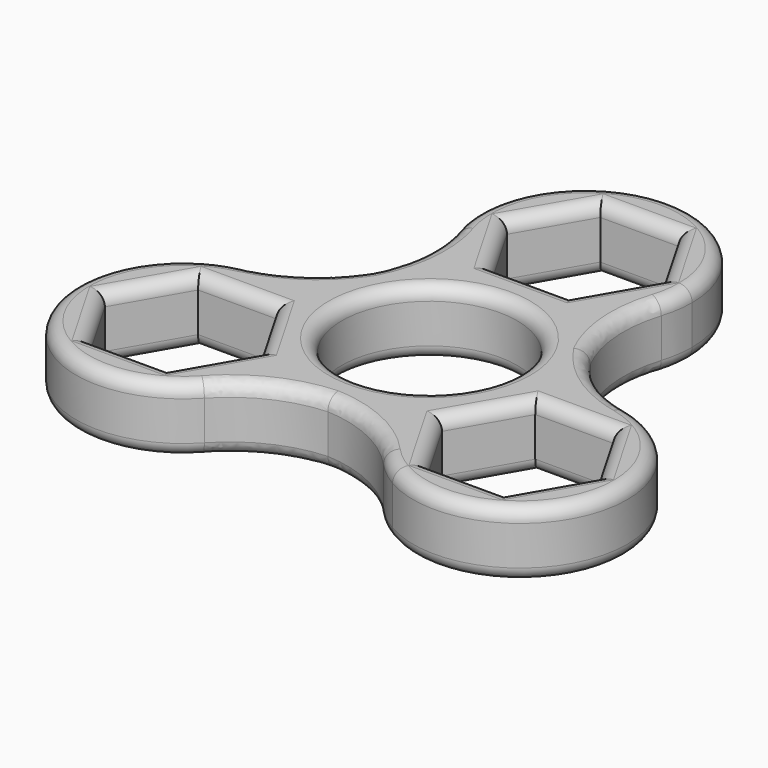
from build123d import *

# Parameters (mm, degrees)
F3_DEPTH = 5
F4_R     = 10
F5_COUNT = 3
F6_R     = 1


# Not quite as in the source:
# - a feature of the source that left no trace in its solid (it failed there, or was rolled back) is left out


with BuildPart() as f3:
    # F2 (on Top) → F3 (new body)
    with BuildSketch(Plane.XY):
        with BuildLine():
            ThreePointArc((8.175, 14.875), (-3.6420010923, 22.193910646), (-4.9299426406, 8.3537815126))
            ThreePointArc((-4.9299426406, 8.3537815126), (-2.5552220381, 9.3573949546), (0, 9.7))
            ThreePointArc((0, 9.7), (2.5552220381, 9.3573949546), (4.9299426406, 8.3537815126))
            ThreePointArc((4.9299426406, 8.3537815126), (7.318910646, 11.2329989077), (8.175, 14.875))
        make_face()
        Polygon((2.9877876431, 9.7), (0, 9.7), (-2.9877876431, 9.7), (-5.9755752861, 14.875), (-2.9877876431, 20.05), (2.9877876431, 20.05), (5.9755752861, 14.875), align=None, mode=Mode.SUBTRACT)
        with BuildLine():
            ThreePointArc((-4.9299426406, 8.3537815126), (-2.5999676792, 7.1244649819), (0, 6.7))
            ThreePointArc((0, 6.7), (2.5999676792, 7.1244649819), (4.9299426406, 8.3537815126))
            ThreePointArc((4.9299426406, 8.3537815126), (2.5552220381, 9.3573949546), (0, 9.7))
            ThreePointArc((0, 9.7), (-2.5552220381, 9.3573949546), (-4.9299426406, 8.3537815126))
        make_face()
        with BuildLine():
            ThreePointArc((4.9299426406, 8.3537815126), (2.5999676792, 7.1244649819), (0, 6.7))
            ThreePointArc((0, 6.7), (-2.5999676792, 7.1244649819), (-4.9299426406, 8.3537815126))
            ThreePointArc((-4.9299426406, 8.3537815126), (-4.8098625961, -8.4234922572), (9.7, 0))
            ThreePointArc((9.7, 0), (8.4234922572, 4.8098625961), (4.9299426406, 8.3537815126))
        make_face()
        with BuildLine():
            ThreePointArc((0, 6.7), (4.7376154339, 4.737615434), (6.7, 0))
            ThreePointArc((6.7, 0), (-4.7376154339, -4.737615434), (0, 6.7))
        make_face(mode=Mode.SUBTRACT)
    extrude(amount=F3_DEPTH)

    # F4
    f4_edges = [f3.edges().sort_by_distance(p)[0] for p in [
        (4.929943, 8.353782, 2.5),
        (-4.929943, 8.353782, 2.5),
    ]]
    fillet(f4_edges, radius=F4_R)

    # F5: F3 ×3 about axis
    f5_axis = Axis((0, 0, 0), (0, 0, -1))


with BuildPart() as f3_1:
    add(f3.part)
    for i in range(1, F5_COUNT):
        add(f3.part.rotate(f5_axis, i * 360 / F5_COUNT))

    # F6
    f6_edges = [f3_1.edges().sort_by_distance(p)[0] for p in [
        (7.357055, 8.567839, 5),
        (0, 23.05, 5),
        (-7.357055, 8.56784, 5),
        (-11.098494, 2.087477, 5),
        (-19.961886, -11.525, 5),
        (-3.741439, -10.655316, 5),
        (3.741439, -10.655316, 5),
        (19.961886, -11.525, 5),
        (11.098494, 2.087477, 5),
        (8.400446, -4.85, 5),
        (12.882128, -2.2625, 5),
        (17.363809, -4.85, 5),
        (17.363809, -10.025, 5),
        (12.882128, -12.6125, 5),
        (8.400446, -10.025, 5),
        (0, 9.7, 5),
        (-4.481681, 12.2875, 5),
        (-4.481681, 17.4625, 5),
        (0, 20.05, 5),
        (4.481681, 17.4625, 5),
        (4.481681, 12.2875, 5),
        (0, -6.7, 5),
        (-12.882128, -12.6125, 5),
        (-17.363809, -10.025, 5),
        (-17.363809, -4.85, 5),
        (-12.882128, -2.2625, 5),
        (-8.400446, -4.85, 5),
        (-8.400446, -10.025, 5),
        (7.357055, 8.567839, 0),
        (0, 23.05, 0),
        (-7.357055, 8.56784, 0),
        (-11.098494, 2.087477, 0),
        (-19.961886, -11.525, 0),
        (-3.741439, -10.655316, 0),
        (3.741439, -10.655316, 0),
        (19.961886, -11.525, 0),
        (11.098494, 2.087477, 0),
        (8.400446, -4.85, 0),
        (12.882128, -2.2625, 0),
        (17.363809, -4.85, 0),
        (17.363809, -10.025, 0),
        (12.882128, -12.6125, 0),
        (8.400446, -10.025, 0),
        (0, 9.7, 0),
        (-4.481681, 12.2875, 0),
        (-4.481681, 17.4625, 0),
        (0, 20.05, 0),
        (4.481681, 17.4625, 0),
        (4.481681, 12.2875, 0),
        (0, -6.7, 0),
        (-12.882128, -12.6125, 0),
        (-17.363809, -10.025, 0),
        (-17.363809, -4.85, 0),
        (-12.882128, -2.2625, 0),
        (-8.400446, -4.85, 0),
        (-8.400446, -10.025, 0),
    ]]
    fillet(f6_edges, radius=F6_R)


solid = f3_1.part
